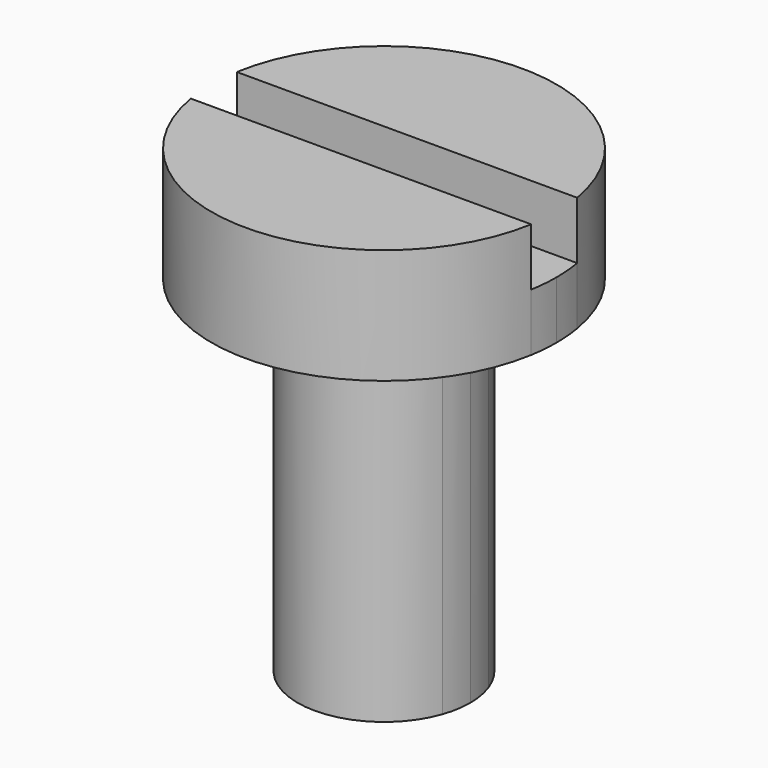
from build123d import *

# Parameters (mm, degrees)
F1_DEPTH = 6
F2_DEPTH = 2
F3_DEPTH = 1


# Not quite as in the source:
# - a feature names something its author has since deleted; it is built from what else it names


with BuildPart() as f1:
    # F0 (on Top) → F1 (new body)
    with BuildSketch(Plane.XY):
        with BuildLine():
            Line((-1.4142135624, 0.5), (1.4142135624, 0.5))
            ThreePointArc((1.4142135624, 0.5), (0, 1.5), (-1.4142135624, 0.5))
        make_face()
        with BuildLine():
            ThreePointArc((1.5, 0), (1.4783978395, 0.2536529681), (1.4142135624, 0.5))
            Line((1.4142135624, 0.5), (-1.4142135624, 0.5))
            ThreePointArc((-1.4142135624, 0.5), (-1.5, 0), (-1.4142135624, -0.5))
            Line((-1.4142135624, -0.5), (1.4142135624, -0.5))
            ThreePointArc((1.4142135624, -0.5), (1.4783978395, -0.2536529681), (1.5, 0))
        make_face()
        with BuildLine():
            ThreePointArc((-1.4142135624, -0.5), (0, -1.5), (1.4142135624, -0.5))
            Line((1.4142135624, -0.5), (-1.4142135624, -0.5))
        make_face()
    extrude(amount=-F1_DEPTH)

    # F0 (on Top) → F2 (join)
    with BuildSketch(Plane.XY):
        with BuildLine():
            ThreePointArc((-2.9580398915, -0.5), (0, -3), (2.9580398915, -0.5))
            Line((2.9580398915, -0.5), (1.4142135624, -0.5))
            ThreePointArc((1.4142135624, -0.5), (0, -1.5), (-1.4142135624, -0.5))
            Line((-1.4142135624, -0.5), (-2.9580398915, -0.5))
        make_face()
        with BuildLine():
            Line((1.4142135624, 0.5), (2.9580398915, 0.5))
            ThreePointArc((2.9580398915, 0.5), (0, 3), (-2.9580398915, 0.5))
            Line((-2.9580398915, 0.5), (-1.4142135624, 0.5))
            ThreePointArc((-1.4142135624, 0.5), (0, 1.5), (1.4142135624, 0.5))
        make_face()
        with BuildLine():
            Line((-1.4142135624, 0.5), (1.4142135624, 0.5))
            ThreePointArc((1.4142135624, 0.5), (0, 1.5), (-1.4142135624, 0.5))
        make_face()
        with BuildLine():
            ThreePointArc((-1.4142135624, -0.5), (0, -1.5), (1.4142135624, -0.5))
            Line((1.4142135624, -0.5), (-1.4142135624, -0.5))
        make_face()
    extrude(amount=F2_DEPTH)

    # F0 (on Top) → F3 (join)
    with BuildSketch(Plane.XY):
        with BuildLine():
            Line((-1.4142135624, 0.5), (-2.9580398915, 0.5))
            ThreePointArc((-2.9580398915, 0.5), (-3, 0), (-2.9580398915, -0.5))
            Line((-2.9580398915, -0.5), (-1.4142135624, -0.5))
            ThreePointArc((-1.4142135624, -0.5), (-1.5, 0), (-1.4142135624, 0.5))
        make_face()
        with BuildLine():
            ThreePointArc((1.5, 0), (1.4783978395, 0.2536529681), (1.4142135624, 0.5))
            Line((1.4142135624, 0.5), (-1.4142135624, 0.5))
            ThreePointArc((-1.4142135624, 0.5), (-1.5, 0), (-1.4142135624, -0.5))
            Line((-1.4142135624, -0.5), (1.4142135624, -0.5))
            ThreePointArc((1.4142135624, -0.5), (1.4783978395, -0.2536529681), (1.5, 0))
        make_face()
        with BuildLine():
            ThreePointArc((2.9580398915, -0.5), (2.9894915684, -0.2508787808), (3, 0))
            ThreePointArc((3, 0), (2.9894915684, 0.2508787808), (2.9580398915, 0.5))
            Line((2.9580398915, 0.5), (1.4142135624, 0.5))
            ThreePointArc((1.4142135624, 0.5), (1.4783978395, 0.2536529681), (1.5, 0))
            ThreePointArc((1.5, 0), (1.4783978395, -0.2536529681), (1.4142135624, -0.5))
            Line((1.4142135624, -0.5), (2.9580398915, -0.5))
        make_face()
    extrude(amount=F3_DEPTH)


solid = f1.part
